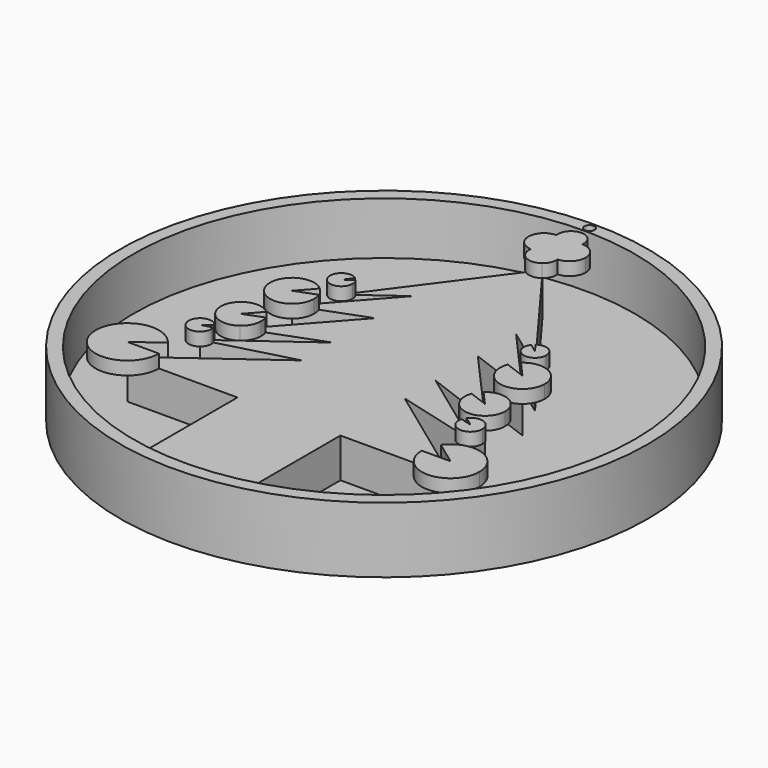
from build123d import *

# Parameters (mm, degrees)
F0_R     = 51.0443252187
F1_DEPTH = 12.7
F2_T     = -2.54
F4_DEPTH = 7.62
F6_DEPTH = 2.54
F7_R     = 0.97697595
F8_DEPTH = 12.701


with BuildPart() as f1:
    # F0 (on Top) → F1 (new body)
    with BuildSketch(Plane.XY):
        Circle(F0_R)
    extrude(amount=F1_DEPTH)

    # F2
    f2_openings = [f1.faces().sort_by_distance(p)[0] for p in [
        (0, 0, 12.7),
    ]]
    offset(amount=F2_T, openings=f2_openings)

    # F3 (on face) → F4 (join)
    with BuildSketch(Plane.XY.offset(2.54)):
        with BuildLine():
            Line((-9.9590039442, -23.0004175437), (-9.9590039442, -47.4709153626))
            ThreePointArc((-9.9590039442, -47.4709153626), (0, -48.5043252187), (9.9590039442, -47.4709153626))
            Line((9.9590039442, -47.4709153626), (9.9590039442, -23.0004175437))
            Line((9.9590039442, -23.0004175437), (31.2569774687, -23.0004175437))
            Line((31.2569774687, -23.0004175437), (9.9590039442, -7.4702212587))
            Line((9.9590039442, -7.4702212587), (26.1457748711, -11.7950867862))
            Line((26.1457748711, -11.7950867862), (9.9590039442, 0))
            Line((9.9590039442, 0), (23.5901717097, -5.1112035289))
            Line((23.5901717097, -5.1112035289), (9.9590039442, 10.2224070579))
            Line((9.9590039442, 10.2224070579), (22.2759793267, 5.6039789728))
            Line((22.2759793267, 5.6039789728), (9.9590039442, 19.4592632281))
            Line((9.9590039442, 19.4592632281), (18.725927211, 13.0709217086))
            Line((18.725927211, 13.0709217086), (0, 38.334030658))
            Line((0, 38.334030658), (-18.725927211, 13.0709217086))
            Line((-18.725927211, 13.0709217086), (-9.9590039442, 19.4592632281))
            Line((-9.9590039442, 19.4592632281), (-22.2759793267, 5.6039789728))
            Line((-22.2759793267, 5.6039789728), (-9.9590039442, 10.2224070579))
            Line((-9.9590039442, 10.2224070579), (-23.5901717097, -5.1112035289))
            Line((-23.5901717097, -5.1112035289), (-9.9590039442, 0))
            Line((-9.9590039442, 0), (-26.1457748711, -11.7950867862))
            Line((-26.1457748711, -11.7950867862), (-9.9590039442, -7.4702212587))
            Line((-9.9590039442, -7.4702212587), (-31.2569774687, -23.0004175437))
            Line((-31.2569774687, -23.0004175437), (-9.9590039442, -23.0004175437))
        make_face()
    extrude(amount=F4_DEPTH)

    # F7 (on face) → F8 (cut, through all)
    with BuildSketch(Plane.XY.offset(12.7)):
        with Locations((0, 49.6633313596)):
            Circle(F7_R)
    extrude(amount=-F8_DEPTH, mode=Mode.SUBTRACT)


with BuildPart() as f6:
    # F5 (on face) → F6 (new body)
    with BuildSketch(Plane.XY.offset(10.16)):
        with BuildLine():
            ThreePointArc((16.9739983826, 14.347529172), (18.0546218787, 11.0097738764), (20.8936405766, 13.0709217086))
            ThreePointArc((20.8936405766, 13.0709217086), (19.7008146252, 15.0070456109), (17.4350875922, 14.8123907189))
            Line((17.4350875922, 14.8123907189), (18.725927211, 13.0709217086))
            Line((18.725927211, 13.0709217086), (16.9739983826, 14.347529172))
        make_face()
    extrude(amount=F6_DEPTH)


with BuildPart() as f6b:
    # F5 (on face) → F6, piece 2 (new body)
    with BuildSketch(Plane.XY.offset(10.16)):
        with BuildLine():
            Line((0.8599322454, 37.1738978773), (1.576613661, 36.2070244895))
            ThreePointArc((1.576613661, 36.2070244895), (2.364754962, 37.1433166508), (2.6476151301, 38.334030658))
            ThreePointArc((2.6476151301, 38.334030658), (2.6439220776, 38.4738230919), (2.6328532228, 38.6132255441))
            ThreePointArc((2.6328532228, 38.6132255441), (1.8888630482, 37.7180710186), (0.8599322454, 37.1738978773))
        make_face()
        with BuildLine():
            ThreePointArc((-1.576613661, 36.2070244895), (0, 35.6864155279), (1.576613661, 36.2070244895))
            Line((1.576613661, 36.2070244895), (0.8599322454, 37.1738978773))
            ThreePointArc((0.8599322454, 37.1738978773), (0, 37.0478709781), (-0.8599322454, 37.1738978773))
            Line((-0.8599322454, 37.1738978773), (-1.576613661, 36.2070244895))
        make_face()
        with BuildLine():
            ThreePointArc((-2.6328532228, 38.6132255441), (-2.4243254196, 37.269835123), (-1.576613661, 36.2070244895))
            Line((-1.576613661, 36.2070244895), (-0.8599322454, 37.1738978773))
            ThreePointArc((-0.8599322454, 37.1738978773), (-1.8888630482, 37.7180710186), (-2.6328532228, 38.6132255441))
        make_face()
        with BuildLine():
            Line((0, 38.334030658), (0.8599322454, 37.1738978773))
            ThreePointArc((0.8599322454, 37.1738978773), (1.8888630482, 37.7180710186), (2.6328532228, 38.6132255441))
            ThreePointArc((2.6328532228, 38.6132255441), (2.6316742989, 38.6241276448), (2.6304502318, 38.6350247691))
            ThreePointArc((2.6304502318, 38.6350247691), (1.110275511, 38.9411279487), (-0.0742141044, 39.9419349677))
            ThreePointArc((-0.0742141044, 39.9419349677), (-1.1966596727, 39.0326567395), (-2.614078781, 38.7540997044))
            ThreePointArc((-2.614078781, 38.7540997044), (-2.6244114093, 38.6837886197), (-2.6328532228, 38.6132255441))
            ThreePointArc((-2.6328532228, 38.6132255441), (-1.8888630482, 37.7180710186), (-0.8599322454, 37.1738978773))
            Line((-0.8599322454, 37.1738978773), (0, 38.334030658))
        make_face()
        with BuildLine():
            ThreePointArc((-0.8599322454, 37.1738978773), (0, 37.0478709781), (0.8599322454, 37.1738978773))
            Line((0.8599322454, 37.1738978773), (0, 38.334030658))
            Line((0, 38.334030658), (-0.8599322454, 37.1738978773))
        make_face()
        with BuildLine():
            ThreePointArc((-2.4592805273, 44.7441331542), (-5.4605012905, 41.8715476694), (-2.7075936217, 38.7601857805))
            ThreePointArc((-2.7075936217, 38.7601857805), (-2.9871101183, 40.2860770487), (-2.4662328709, 41.7472958987))
            ThreePointArc((-2.4662328709, 41.7472958987), (-2.6251055728, 42.9375271186), (-2.2398557502, 44.0748368681))
            ThreePointArc((-2.2398557502, 44.0748368681), (-2.3732803918, 44.4017110911), (-2.4592805273, 44.7441331542))
        make_face()
        with BuildLine():
            ThreePointArc((-2.4662328709, 41.7472958987), (-2.9871101183, 40.2860770487), (-2.7075936217, 38.7601857805))
            ThreePointArc((-2.7075936217, 38.7601857805), (-2.6608599921, 38.7567771888), (-2.614078781, 38.7540997044))
            ThreePointArc((-2.614078781, 38.7540997044), (-2.2383831472, 39.7480698241), (-1.5021368627, 40.5142716361))
            ThreePointArc((-1.5021368627, 40.5142716361), (-2.0777576359, 41.057619649), (-2.4662328709, 41.7472958987))
        make_face()
        with BuildLine():
            ThreePointArc((-1.5021368627, 40.5142716361), (-2.2383831472, 39.7480698241), (-2.614078781, 38.7540997044))
            ThreePointArc((-2.614078781, 38.7540997044), (-1.1966596727, 39.0326567395), (-0.0742141044, 39.9419349677))
            ThreePointArc((-0.0742141044, 39.9419349677), (-0.1110994221, 39.9949953603), (-0.1468766842, 40.0488091079))
            ThreePointArc((-0.1468766842, 40.0488091079), (-0.8567235615, 40.1877366237), (-1.5021368627, 40.5142716361))
        make_face()
        with BuildLine():
            ThreePointArc((2.6304502318, 38.6350247691), (2.6377340362, 38.6354176434), (2.6450169011, 38.6358275643))
            ThreePointArc((2.6450169011, 38.6358275643), (2.9075581156, 39.3186393908), (2.9968453198, 40.0447162979))
            ThreePointArc((2.9968453198, 40.0447162979), (2.8611186892, 40.9363898464), (2.4662328709, 41.7472958987))
            ThreePointArc((2.4662328709, 41.7472958987), (2.0777576359, 41.057619649), (1.5021368627, 40.5142716361))
            ThreePointArc((1.5021368627, 40.5142716361), (2.2699033504, 39.6968969966), (2.6304502318, 38.6350247691))
        make_face()
        with BuildLine():
            ThreePointArc((2.9968453198, 40.0447162979), (2.9075581156, 39.3186393908), (2.6450169011, 38.6358275643))
            ThreePointArc((2.6450169011, 38.6358275643), (4.7323305443, 39.6076697023), (5.5828334109, 41.7472958987))
            ThreePointArc((5.5828334109, 41.7472958987), (4.6739855016, 43.9470748075), (2.4775093982, 44.8638760382))
            ThreePointArc((2.4775093982, 44.8638760382), (2.3914491817, 44.4594873566), (2.2398557502, 44.0748368681))
            ThreePointArc((2.2398557502, 44.0748368681), (2.5361357873, 43.4063510394), (2.6374925045, 42.6822088024))
            ThreePointArc((2.6374925045, 42.6822088024), (2.5943243265, 42.2069741237), (2.4662328709, 41.7472958987))
            ThreePointArc((2.4662328709, 41.7472958987), (2.8611186892, 40.9363898464), (2.9968453198, 40.0447162979))
        make_face()
        with BuildLine():
            ThreePointArc((-0.0742141044, 39.9419349677), (1.110275511, 38.9411279487), (2.6304502318, 38.6350247691))
            ThreePointArc((2.6304502318, 38.6350247691), (2.2699033504, 39.6968969966), (1.5021368627, 40.5142716361))
            ThreePointArc((1.5021368627, 40.5142716361), (0.7869080902, 40.1648406592), (0, 40.0447162979))
            ThreePointArc((0, 40.0447162979), (-0.0365635017, 39.9929331577), (-0.0742141044, 39.9419349677))
        make_face()
        with BuildLine():
            ThreePointArc((-0.9725766756, 42.879354984), (-1.8101773995, 42.4330922426), (-2.4662328709, 41.7472958987))
            ThreePointArc((-2.4662328709, 41.7472958987), (-2.0777576359, 41.057619649), (-1.5021368627, 40.5142716361))
            ThreePointArc((-1.5021368627, 40.5142716361), (-1.04170417, 40.7681050815), (-0.540192524, 40.9259523223))
            ThreePointArc((-0.540192524, 40.9259523223), (-0.6492138876, 41.832092248), (-0.491063748, 42.7309602894))
            ThreePointArc((-0.491063748, 42.7309602894), (-0.7355719331, 42.7929840054), (-0.9725766756, 42.879354984))
        make_face()
        with BuildLine():
            ThreePointArc((-2.2398557502, 44.0748368681), (-2.6251055728, 42.9375271186), (-2.4662328709, 41.7472958987))
            ThreePointArc((-2.4662328709, 41.7472958987), (-1.8101773995, 42.4330922426), (-0.9725766756, 42.879354984))
            ThreePointArc((-0.9725766756, 42.879354984), (-1.7138333514, 43.363015613), (-2.2398557502, 44.0748368681))
        make_face()
        with BuildLine():
            ThreePointArc((-1.7484128812, 44.6569034897), (-2.1012315183, 44.7218304646), (-2.4592805273, 44.7441331542))
            ThreePointArc((-2.4592805273, 44.7441331542), (-2.3732803918, 44.4017110911), (-2.2398557502, 44.0748368681))
            ThreePointArc((-2.2398557502, 44.0748368681), (-2.0152597989, 44.3837065703), (-1.7484128812, 44.6569034897))
        make_face()
        with BuildLine():
            ThreePointArc((2.497568045, 45.1797768474), (-0.2186614743, 47.6677546003), (-2.4592805273, 44.7441331542))
            ThreePointArc((-2.4592805273, 44.7441331542), (-2.1012315183, 44.7218304646), (-1.7484128812, 44.6569034897))
            ThreePointArc((-1.7484128812, 44.6569034897), (-0.0734668488, 45.3186779058), (1.6357329288, 44.7512048141))
            ThreePointArc((1.6357329288, 44.7512048141), (2.052765276, 44.8363480954), (2.4775093982, 44.8638760382))
            ThreePointArc((2.4775093982, 44.8638760382), (2.4925483389, 45.0215083488), (2.497568045, 45.1797768474))
        make_face()
        with BuildLine():
            ThreePointArc((-0.540192524, 40.9259523223), (-1.04170417, 40.7681050815), (-1.5021368627, 40.5142716361))
            ThreePointArc((-1.5021368627, 40.5142716361), (-0.8567235615, 40.1877366237), (-0.1468766842, 40.0488091079))
            ThreePointArc((-0.1468766842, 40.0488091079), (-0.3775565584, 40.4721250838), (-0.540192524, 40.9259523223))
        make_face()
        with BuildLine():
            ThreePointArc((0.421999424, 40.947798506), (0.986185327, 40.7911233257), (1.5021368627, 40.5142716361))
            ThreePointArc((1.5021368627, 40.5142716361), (2.0777576359, 41.057619649), (2.4662328709, 41.7472958987))
            ThreePointArc((2.4662328709, 41.7472958987), (1.8101773995, 42.4330922426), (0.9725766756, 42.879354984))
            ThreePointArc((0.9725766756, 42.879354984), (0.677480511, 42.7758495822), (0.3717630065, 42.7100322439))
            ThreePointArc((0.3717630065, 42.7100322439), (0.4906334207, 42.2351725265), (0.5306124489, 41.7472958987))
            ThreePointArc((0.5306124489, 41.7472958987), (0.5033350527, 41.3438752528), (0.421999424, 40.947798506))
        make_face()
        with BuildLine():
            ThreePointArc((0, 40.0447162979), (0.7869080902, 40.1648406592), (1.5021368627, 40.5142716361))
            ThreePointArc((1.5021368627, 40.5142716361), (0.986185327, 40.7911233257), (0.421999424, 40.947798506))
            ThreePointArc((0.421999424, 40.947798506), (0.248811083, 40.4785886043), (0, 40.0447162979))
        make_face()
        with BuildLine():
            ThreePointArc((-1.7484128812, 44.6569034897), (-2.0152597989, 44.3837065703), (-2.2398557502, 44.0748368681))
            ThreePointArc((-2.2398557502, 44.0748368681), (-1.7138333514, 43.363015613), (-0.9725766756, 42.879354984))
            ThreePointArc((-0.9725766756, 42.879354984), (-0.6797144374, 42.9634609175), (-0.3798256388, 43.0173942749))
            ThreePointArc((-0.3798256388, 43.0173942749), (-0.2402846028, 43.2925991344), (-0.0742141044, 43.5526568298))
            ThreePointArc((-0.0742141044, 43.5526568298), (-0.8161981913, 44.2489888109), (-1.7484128812, 44.6569034897))
        make_face()
        with BuildLine():
            ThreePointArc((-0.3798256388, 43.0173942749), (-0.6797144374, 42.9634609175), (-0.9725766756, 42.879354984))
            ThreePointArc((-0.9725766756, 42.879354984), (-0.7355719331, 42.7929840054), (-0.491063748, 42.7309602894))
            ThreePointArc((-0.491063748, 42.7309602894), (-0.4389768968, 42.8755490315), (-0.3798256388, 43.0173942749))
        make_face()
        with BuildLine():
            ThreePointArc((1.6357329288, 44.7512048141), (-0.0734668488, 45.3186779058), (-1.7484128812, 44.6569034897))
            ThreePointArc((-1.7484128812, 44.6569034897), (-0.8161981913, 44.2489888109), (-0.0742141044, 43.5526568298))
            ThreePointArc((-0.0742141044, 43.5526568298), (0.6773924371, 44.2994026418), (1.6357329288, 44.7512048141))
        make_face()
        with BuildLine():
            ThreePointArc((-0.540192524, 40.9259523223), (-0.3775565584, 40.4721250838), (-0.1468766842, 40.0488091079))
            ThreePointArc((-0.1468766842, 40.0488091079), (-0.0734668488, 40.045739699), (0, 40.0447162979))
            ThreePointArc((0, 40.0447162979), (0.248811083, 40.4785886043), (0.421999424, 40.947798506))
            ThreePointArc((0.421999424, 40.947798506), (-0.0600975553, 40.9809636305), (-0.540192524, 40.9259523223))
        make_face()
        with BuildLine():
            ThreePointArc((-0.491063748, 42.7309602894), (-0.6492138876, 41.832092248), (-0.540192524, 40.9259523223))
            ThreePointArc((-0.540192524, 40.9259523223), (-0.0600975553, 40.9809636305), (0.421999424, 40.947798506))
            ThreePointArc((0.421999424, 40.947798506), (0.5033350527, 41.3438752528), (0.5306124489, 41.7472958987))
            ThreePointArc((0.5306124489, 41.7472958987), (0.4906334207, 42.2351725265), (0.3717630065, 42.7100322439))
            ThreePointArc((0.3717630065, 42.7100322439), (-0.0605612294, 42.6829431571), (-0.491063748, 42.7309602894))
        make_face()
        with BuildLine():
            ThreePointArc((0.9725766756, 42.879354984), (1.8101773995, 42.4330922426), (2.4662328709, 41.7472958987))
            ThreePointArc((2.4662328709, 41.7472958987), (2.5943243265, 42.2069741237), (2.6374925045, 42.6822088024))
            ThreePointArc((2.6374925045, 42.6822088024), (2.5361357873, 43.4063510394), (2.2398557502, 44.0748368681))
            ThreePointArc((2.2398557502, 44.0748368681), (1.7138333514, 43.363015613), (0.9725766756, 42.879354984))
        make_face()
        with BuildLine():
            ThreePointArc((2.2398557502, 44.0748368681), (2.3914491817, 44.4594873566), (2.4775093982, 44.8638760382))
            ThreePointArc((2.4775093982, 44.8638760382), (2.052765276, 44.8363480954), (1.6357329288, 44.7512048141))
            ThreePointArc((1.6357329288, 44.7512048141), (1.9670829423, 44.4391810302), (2.2398557502, 44.0748368681))
        make_face()
        with BuildLine():
            ThreePointArc((-0.3798256388, 43.0173942749), (-0.4389768968, 42.8755490315), (-0.491063748, 42.7309602894))
            ThreePointArc((-0.491063748, 42.7309602894), (-0.0605612294, 42.6829431571), (0.3717630065, 42.7100322439))
            ThreePointArc((0.3717630065, 42.7100322439), (0.3112261469, 42.8728194547), (0.2413607508, 43.0318264162))
            ThreePointArc((0.2413607508, 43.0318264162), (-0.0696074922, 43.0407531248), (-0.3798256388, 43.0173942749))
        make_face()
        with BuildLine():
            ThreePointArc((-0.0742141044, 43.5526568298), (-0.2402846028, 43.2925991344), (-0.3798256388, 43.0173942749))
            ThreePointArc((-0.3798256388, 43.0173942749), (-0.0696074922, 43.0407531248), (0.2413607508, 43.0318264162))
            ThreePointArc((0.2413607508, 43.0318264162), (0.0968371062, 43.3002782435), (-0.0742141044, 43.5526568298))
        make_face()
        with BuildLine():
            ThreePointArc((2.2398557502, 44.0748368681), (1.9670829423, 44.4391810302), (1.6357329288, 44.7512048141))
            ThreePointArc((1.6357329288, 44.7512048141), (0.6773924371, 44.2994026418), (-0.0742141044, 43.5526568298))
            ThreePointArc((-0.0742141044, 43.5526568298), (0.0968371062, 43.3002782435), (0.2413607508, 43.0318264162))
            ThreePointArc((0.2413607508, 43.0318264162), (0.6117376098, 42.9784611688), (0.9725766756, 42.879354984))
            ThreePointArc((0.9725766756, 42.879354984), (1.7138333514, 43.363015613), (2.2398557502, 44.0748368681))
        make_face()
        with BuildLine():
            ThreePointArc((0.3717630065, 42.7100322439), (0.677480511, 42.7758495822), (0.9725766756, 42.879354984))
            ThreePointArc((0.9725766756, 42.879354984), (0.6117376098, 42.9784611688), (0.2413607508, 43.0318264162))
            ThreePointArc((0.2413607508, 43.0318264162), (0.3112261469, 42.8728194547), (0.3717630065, 42.7100322439))
        make_face()
    extrude(amount=F6_DEPTH)


with BuildPart() as f6c:
    # F5 (on face) → F6, piece 3 (new body)
    with BuildSketch(Plane.XY.offset(10.16)):
        with BuildLine():
            ThreePointArc((26.5862698893, 5.6039789728), (24.0416234273, 9.536040219), (19.4122265529, 8.8253955532))
            Line((19.4122265529, 8.8253955532), (22.2759793267, 5.6039789728))
            Line((22.2759793267, 5.6039789728), (18.2400813608, 7.1172972945))
            ThreePointArc((18.2400813608, 7.1172972945), (21.5069826362, 1.3628412924), (26.5862698893, 5.6039789728))
        make_face()
    extrude(amount=F6_DEPTH)


with BuildPart() as f6d:
    # F5 (on face) → F6, piece 4 (new body)
    with BuildSketch(Plane.XY.offset(10.16)):
        with BuildLine():
            Line((-18.725927211, 13.0709217086), (-17.4350875922, 14.8123907189))
            ThreePointArc((-17.4350875922, 14.8123907189), (-20.6620511133, 12.0960342944), (-16.5582138454, 13.0709217086))
            ThreePointArc((-16.5582138454, 13.0709217086), (-16.6647793788, 13.742227041), (-16.9739983826, 14.347529172))
            Line((-16.9739983826, 14.347529172), (-18.725927211, 13.0709217086))
        make_face()
    extrude(amount=F6_DEPTH)


with BuildPart() as f6e:
    # F5 (on face) → F6, piece 5 (new body)
    with BuildSketch(Plane.XY.offset(10.16)):
        with BuildLine():
            ThreePointArc((27.4922685848, -5.1112035289), (25.1886055571, -1.5515168491), (20.9976224168, -2.194861953))
            Line((20.9976224168, -2.194861953), (23.5901717097, -5.1112035289))
            Line((23.5901717097, -5.1112035289), (19.9364818684, -3.7411996722))
            ThreePointArc((19.9364818684, -3.7411996722), (19.8244494224, -6.1337961548), (21.1312859186, -8.1410947299))
            Line((21.1312859186, -8.1410947299), (21.4592369578, -8.3800683329))
            ThreePointArc((21.4592369578, -8.3800683329), (25.4491023414, -8.5420542878), (27.4922685848, -5.1112035289))
        make_face()
    extrude(amount=F6_DEPTH)


with BuildPart() as f6f:
    # F5 (on face) → F6, piece 6 (new body)
    with BuildSketch(Plane.XY.offset(10.16)):
        with BuildLine():
            Line((-22.2759793267, 5.6039789728), (-19.4507515767, 8.7820590084))
            ThreePointArc((-19.4507515767, 8.7820590084), (-26.1551439841, 3.8620874397), (-18.0236735343, 5.6039789728))
            ThreePointArc((-18.0236735343, 5.6039789728), (-18.091896128, 6.3626306306), (-18.2943748273, 7.0969391739))
            Line((-18.2943748273, 7.0969391739), (-22.2759793267, 5.6039789728))
        make_face()
    extrude(amount=F6_DEPTH)


with BuildPart() as f6g:
    # F5 (on face) → F6, piece 7 (new body)
    with BuildSketch(Plane.XY.offset(10.16)):
        with BuildLine():
            ThreePointArc((28.4383269565, -11.7950867862), (26.8557407107, -9.6152373485), (24.2929523749, -10.4449594358))
            Line((24.2929523749, -10.4449594358), (26.1457748711, -11.7950867862))
            Line((26.1457748711, -11.7950867862), (23.9309171294, -11.2033095912))
            ThreePointArc((23.9309171294, -11.2033095912), (25.8473470492, -14.0681322981), (28.4383269565, -11.7950867862))
        make_face()
    extrude(amount=F6_DEPTH)


with BuildPart() as f6h:
    # F5 (on face) → F6, piece 8 (new body)
    with BuildSketch(Plane.XY.offset(10.16)):
        with BuildLine():
            Line((-23.5901717097, -5.1112035289), (-21.0011293185, -2.1988068435))
            ThreePointArc((-21.0011293185, -2.1988068435), (-27.4824109739, -4.9223425581), (-21.2952614562, -8.2605815445))
            ThreePointArc((-21.2952614562, -8.2605815445), (-20.1168416184, -6.8778877208), (-19.6933531411, -5.1112035289))
            ThreePointArc((-19.6933531411, -5.1112035289), (-19.7558724148, -4.4159741612), (-19.9414241586, -3.7430528554))
            Line((-19.9414241586, -3.7430528554), (-23.5901717097, -5.1112035289))
        make_face()
    extrude(amount=F6_DEPTH)


with BuildPart() as f6i:
    # F5 (on face) → F6, piece 9 (new body)
    with BuildSketch(Plane.XY.offset(10.16)):
        with BuildLine():
            Line((-26.1457748711, -11.7950867862), (-24.3694626867, -10.5007114924))
            ThreePointArc((-24.3694626867, -10.5007114924), (-28.2356097712, -12.4757353502), (-23.9478912578, -11.7950867862))
            ThreePointArc((-23.9478912578, -11.7950867862), (-23.9665923283, -11.5089822201), (-24.0223772972, -11.2277463938))
            Line((-24.0223772972, -11.2277463938), (-26.1457748711, -11.7950867862))
        make_face()
    extrude(amount=F6_DEPTH)


with BuildPart() as f6j:
    # F5 (on face) → F6, piece 10 (new body)
    with BuildSketch(Plane.XY.offset(10.16)):
        with BuildLine():
            ThreePointArc((36.8241791531, -23.0004175437), (32.981912388, -17.7071827937), (26.75867921, -19.7203188608))
            Line((26.75867921, -19.7203188608), (31.2569774687, -23.0004175437))
            Line((31.2569774687, -23.0004175437), (25.6897757844, -23.0004175437))
            ThreePointArc((25.6897757844, -23.0004175437), (31.2569774687, -28.567619228), (36.8241791531, -23.0004175437))
        make_face()
    extrude(amount=F6_DEPTH)


with BuildPart() as f6k:
    # F5 (on face) → F6, piece 11 (new body)
    with BuildSketch(Plane.XY.offset(10.16)):
        with BuildLine():
            Line((-31.2569774687, -23.0004175437), (-26.3099207792, -19.3930902394))
            ThreePointArc((-26.3099207792, -19.3930902394), (-37.0782749624, -24.8974351136), (-25.1343816002, -23.0004175437))
            Line((-25.1343816002, -23.0004175437), (-31.2569774687, -23.0004175437))
        make_face()
    extrude(amount=F6_DEPTH)


solid = Compound([f1.part, f6.part, f6b.part, f6c.part, f6d.part, f6e.part, f6f.part, f6g.part, f6h.part, f6i.part, f6j.part, f6k.part])
